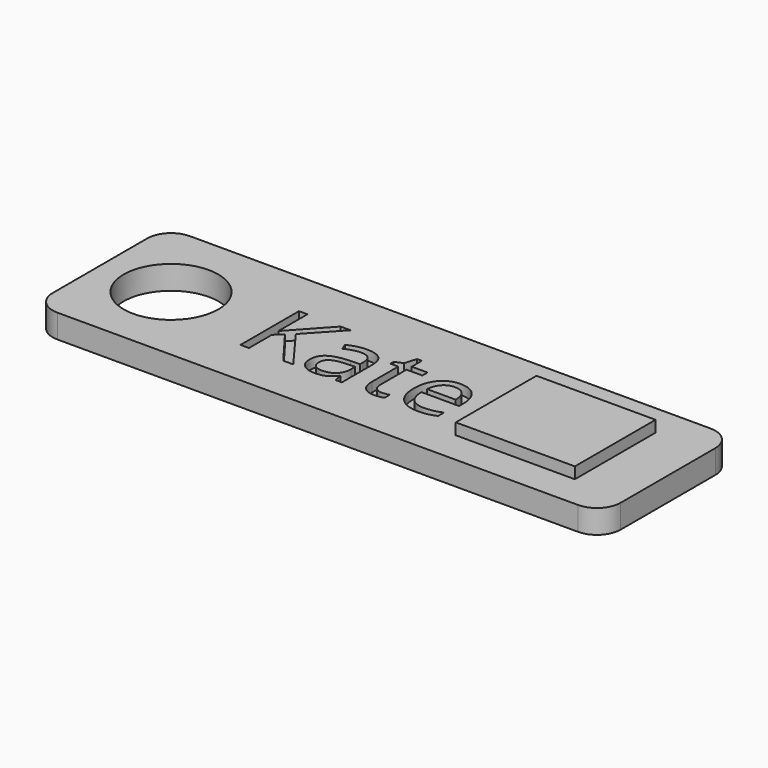
from build123d import *

# Parameters (mm, degrees)
F0_W         = 120
F0_H         = 35
F0_R         = 10
F1_DEPTH     = 5
F2_R         = 5
F3_R         = 5
F4_R         = 5
F7_R         = 5
F5_TEXT_SIZE = 21.6288133136
F8_DEPTH     = 2
F9_W         = 25.1644738019
F9_H         = 21.3157907128
F10_DEPTH    = 2.4


# Not quite as in the source:
# - Text() gives the source's letters only with a copy of the font that has no kerning and outlines rounded to 1/6400 em; it was checked with that copy


with BuildPart() as f1:
    # F0 (on Top) → F1 (new body)
    with BuildSketch(Plane.XY):
        Rectangle(F0_W, F0_H)
        with Locations((-45, 0)):
            Circle(F0_R, mode=Mode.SUBTRACT)
    extrude(amount=F1_DEPTH)

    # F2
    f2_edges = [f1.edges().sort_by_distance(p)[0] for p in [
        (60, -17.5, 2.5),
    ]]
    fillet(f2_edges, radius=F2_R)

    # F3
    f3_edges = [f1.edges().sort_by_distance(p)[0] for p in [
        (60, 17.5, 2.5),
    ]]
    fillet(f3_edges, radius=F3_R)

    # F4
    f4_edges = [f1.edges().sort_by_distance(p)[0] for p in [
        (-60, -17.5, 2.5),
    ]]
    fillet(f4_edges, radius=F4_R)

    # F7
    f7_edges = [f1.edges().sort_by_distance(p)[0] for p in [
        (-60, 17.5, 2.5),
    ]]
    fillet(f7_edges, radius=F7_R)

    # F5 (on face) → F8 (cut)
    with BuildSketch(Plane.XY.offset(5)):
        with Locations((-26.344390586, -7.6336544007)):
            Text('Kate', F5_TEXT_SIZE, font='Open Sans', text_align=(TextAlign.LEFT, TextAlign.BOTTOM))
    extrude(amount=-F8_DEPTH, mode=Mode.SUBTRACT)

    # F9 (on face) → F10 (join)
    with BuildSketch(Plane.XY.offset(5)):
        with Locations((36.2664479762, 0)):
            Rectangle(F9_W, F9_H)
    extrude(amount=F10_DEPTH)


solid = f1.part
